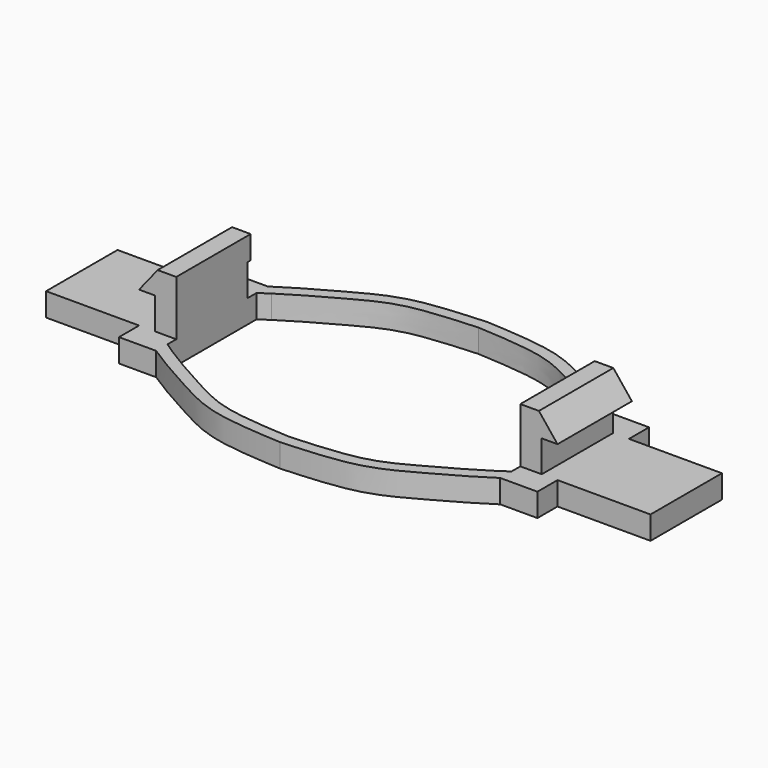
from build123d import *

# Parameters (mm, degrees)
F1_DEPTH = 2.5
F2_W     = 2.3
F2_H     = 9.6
F3_DEPTH = 3.4
F5_DEPTH = 10


# Not quite as in the source:
# - ends of sketch curves that miss each other by under 0.0002 mm in the source are joined
# - the dataset's text gives a spline's control points without its knots; the knots are read off the source's solid


with BuildPart() as f1:
    # F0 (on Top) → F1 (new body)
    with BuildSketch(Plane.XY):
        with BuildLine():
            Line((32.5, -4.8), (32.5, 0))
            Line((32.5, 0), (32.5, 4.8))
            Line((32.5, 4.8), (22.5, 4.8))
            Line((22.5, 4.8), (22.5, 7.5))
            Line((22.5, 7.5), (18.5, 7.5))
            add(Edge.make_bspline(
                [(18.5, 7.5), (16.6328875571, 8.7478424674), (12.4879926615, 11.0335251601), (7.8863773573, 13.5145464122), (2.5994103613, 13.8122400643), (0, 13.9694881193)],
                knots=[0, 0, 0, 0, 0.3363717727, 0.6336483956, 0.9777931055, 0.9777931055, 0.9777931055, 0.9777931055], degree=3))
            add(Edge.make_bspline(
                [(-18.5, 7.5), (-16.6328875571, 8.7478424674), (-12.4879926615, 11.0335251601), (-7.8863773573, 13.5145464122), (-2.5994103613, 13.8122400643), (0, 13.9694881193)],
                knots=[0, 0, 0, 0, 0.3363717727, 0.6336483956, 0.9777931055, 0.9777931055, 0.9777931055, 0.9777931055], degree=3))
            Line((-18.5, 7.5), (-22.5, 7.5))
            Line((-22.5, 7.5), (-22.5, 4.8))
            Line((-22.5, 4.8), (-32.5, 4.8))
            Line((-32.5, 4.8), (-32.5, 0))
            Line((-32.5, 0), (-32.5, -4.8))
            Line((-32.5, -4.8), (-22.5, -4.8))
            Line((-22.5, -4.8), (-22.5, -7.5))
            Line((-22.5, -7.5), (-18.5, -7.5))
            add(Edge.make_bspline(
                [(-18.5, -7.5), (-16.6328875571, -8.7478424674), (-12.4879926615, -11.0335251601), (-7.8863773573, -13.5145464122), (-2.5994103613, -13.8122400643), (0, -13.9694881193)],
                knots=[0, 0, 0, 0, 0.3363717727, 0.6336483956, 0.9777931055, 0.9777931055, 0.9777931055, 0.9777931055], degree=3))
            add(Edge.make_bspline(
                [(18.5, -7.5), (16.6328875571, -8.7478424674), (12.4879926615, -11.0335251601), (7.8863773573, -13.5145464122), (2.5994103613, -13.8122400643), (0, -13.9694881193)],
                knots=[0, 0, 0, 0, 0.3363717727, 0.6336483956, 0.9777931055, 0.9777931055, 0.9777931055, 0.9777931055], degree=3))
            Line((18.5, -7.5), (22.5, -7.5))
            Line((22.5, -7.5), (22.5, -4.8))
            Line((22.5, -4.8), (32.5, -4.8))
        make_face()
        with BuildLine():
            Line((-18.5, 0), (-18.5, 5.9768469073))
            Line((-18.5, 5.9768469073), (-17.4557828979, 6.6914400202))
            add(Edge.make_bspline(
                [(-17.4557828979, 6.6914400202), (-16.8874977541, 7.0617589277), (-15.5631242254, 7.8773690533), (-13.8072733089, 8.8734333253), (-12.5364597536, 9.5720832259), (-11.8350717008, 9.9552778211), (-11.1621909622, 10.3213808687), (-10.364996594, 10.7418634519), (-9.4382542316, 11.1823324733), (-8.4958782817, 11.5579825068), (-7.6562822144, 11.8178001131), (-6.921672188, 11.9930107338), (-6.1338774618, 12.1498095188), (-5.0696801932, 12.3116557143), (-3.7025355233, 12.4602871457), (-2.0018671704, 12.5972327818), (-0.7534045854, 12.6716577772), (5.394e-07, 12.717197038)],
                knots=[0.0214889286, 0.0214889286, 0.0214889286, 0.0214889286, 0.125, 0.25, 0.3125, 0.34375, 0.375, 0.4375, 0.5, 0.5625, 0.625, 0.65625, 0.6875, 0.75, 0.8125, 0.875, 0.9744706617, 0.9744706617, 0.9744706617, 0.9744706617], degree=3))
            add(Edge.make_bspline(
                [(17.4557781808, 6.6914327816), (16.8874977541, 7.0617589277), (15.5631242254, 7.8773690533), (13.8072733089, 8.8734333253), (12.5364597536, 9.5720832259), (11.8350717008, 9.9552778211), (11.1621909622, 10.3213808687), (10.364996594, 10.7418634519), (9.4382542316, 11.1823324733), (8.4958782817, 11.5579825068), (7.6562822144, 11.8178001131), (6.921672188, 11.9930107338), (6.1338774618, 12.1498095188), (5.0696801932, 12.3116557143), (3.7025355233, 12.4602871457), (2.0018675288, 12.597232753), (0.7534053146, 12.6716577338), (5.394e-07, 12.717197038)],
                knots=[0.0214889286, 0.0214889286, 0.0214889286, 0.0214889286, 0.125, 0.25, 0.3125, 0.34375, 0.375, 0.4375, 0.5, 0.5625, 0.625, 0.65625, 0.6875, 0.75, 0.8125, 0.875, 0.9744706144, 0.9744706144, 0.9744706144, 0.9744706144], degree=3))
            Line((17.4557781808, 6.6914327816), (18.5, 5.9768469073))
            Line((18.5, 5.9768469073), (18.5, 5))
            Line((18.5, 5), (18.5, 0))
            Line((18.5, 0), (18.5, -5.9768469073))
            Line((18.5, -5.9768469073), (17.4557828979, -6.6914400202))
            add(Edge.make_bspline(
                [(17.4557828979, -6.6914400202), (16.8874977541, -7.0617589277), (15.5631242254, -7.8773690533), (13.8072733089, -8.8734333253), (12.5364597536, -9.5720832259), (11.8350717008, -9.9552778211), (11.1621909622, -10.3213808687), (10.364996594, -10.7418634519), (9.4382542316, -11.1823324733), (8.4958782817, -11.5579825068), (7.6562822144, -11.8178001131), (6.921672188, -11.9930107338), (6.1338774618, -12.1498095188), (5.0696801932, -12.3116557143), (3.7025355233, -12.4602871457), (2.0018673502, -12.5972327673), (0.7534049513, -12.6716577554), (0, -12.7171970054)],
                knots=[0.0214889286, 0.0214889286, 0.0214889286, 0.0214889286, 0.125, 0.25, 0.3125, 0.34375, 0.375, 0.4375, 0.5, 0.5625, 0.625, 0.65625, 0.6875, 0.75, 0.8125, 0.875, 0.974470638, 0.974470638, 0.974470638, 0.974470638], degree=3))
            add(Edge.make_bspline(
                [(-17.4557781808, -6.6914327816), (-16.8874977541, -7.0617589277), (-15.5631242254, -7.8773690533), (-13.8072733089, -8.8734333253), (-12.5364597536, -9.5720832259), (-11.8350717008, -9.9552778211), (-11.1621909622, -10.3213808687), (-10.364996594, -10.7418634519), (-9.4382542316, -11.1823324733), (-8.4958782817, -11.5579825068), (-7.6562822144, -11.8178001131), (-6.921672188, -11.9930107338), (-6.1338774618, -12.1498095188), (-5.0696801932, -12.3116557143), (-3.7025355233, -12.4602871457), (-2.0018673502, -12.5972327673), (-0.7534049513, -12.6716577554), (0, -12.7171970054)],
                knots=[0.0214889286, 0.0214889286, 0.0214889286, 0.0214889286, 0.125, 0.25, 0.3125, 0.34375, 0.375, 0.4375, 0.5, 0.5625, 0.625, 0.65625, 0.6875, 0.75, 0.8125, 0.875, 0.974470638, 0.974470638, 0.974470638, 0.974470638], degree=3))
            Line((-17.4557781808, -6.6914327816), (-18.5, -5.9768469073))
            Line((-18.5, -5.9768469073), (-18.5, 0))
        make_face(mode=Mode.SUBTRACT)
    extrude(amount=-F1_DEPTH)

    # F2 (on face) → F3 (join)
    with BuildSketch(Plane.XY):
        with Locations((19.65, 0)):
            Rectangle(F2_W, F2_H)
        with Locations((-19.65, 0)):
            Rectangle(F2_W, F2_H)
    extrude(amount=F3_DEPTH)

    # F4 (on face) → F5 (join)
    with BuildSketch(Plane.XZ.offset(4.8)):
        Polygon((18.5, 5.9), (18.5, 3.4), (22.5, 3.4), (20.5, 5.9), align=None)
        Polygon((-20.5, 5.9), (-22.5, 3.4), (-18.5, 3.4), (-18.5, 5.9), align=None)
    extrude(amount=-F5_DEPTH)


solid = f1.part
